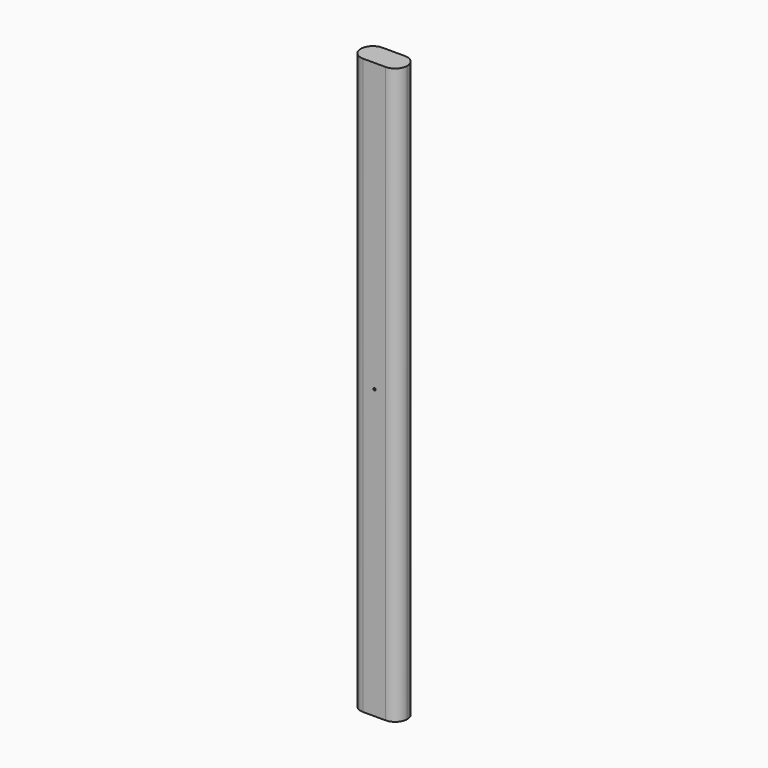
from build123d import *

# Parameters (mm, degrees)
F0_W     = 196.85
F0_H     = 101.6
F1_DEPTH = 2438.4
F2_R     = 50.79999
F3_R     = 4.7625
F4_DEPTH = 25.4
F5_DEPTH = 25.4


# Not quite as in the source:
# - a fillet or chamfer is up to 0.001 mm smaller than in the source, because OpenCascade refuses the exact size


with BuildPart() as f1:
    # F0 (on Top) → F1 (new body)
    with BuildSketch(Plane.XY):
        with Locations((-98.425, 50.8)):
            Rectangle(F0_W, F0_H)
    extrude(amount=F1_DEPTH)

    # F2 (radius 50.8 in the source; OpenCascade refuses exactly that, so slightly less here)
    f2_edges = [f1.edges().sort_by_distance(p)[0] for p in [
        (0, 0, 1219.2),
        (-196.85, 0, 1219.2),
        (-196.85, 101.6, 1219.2),
        (0, 101.6, 1219.2),
    ]]
    fillet(f2_edges, radius=F2_R)

    # F3 (on face) → F4 (cut)
    with BuildSketch(Plane.XZ):
        with Locations((-98.425, 1220.7875)):
            Circle(F3_R)
    extrude(amount=-F4_DEPTH, mode=Mode.SUBTRACT)

    # F3 (on face) → F5 (cut)
    with BuildSketch(Plane.XZ):
        with Locations((-98.425, 1220.7875)):
            Circle(F3_R)
    extrude(amount=-F5_DEPTH, mode=Mode.SUBTRACT)


solid = f1.part
